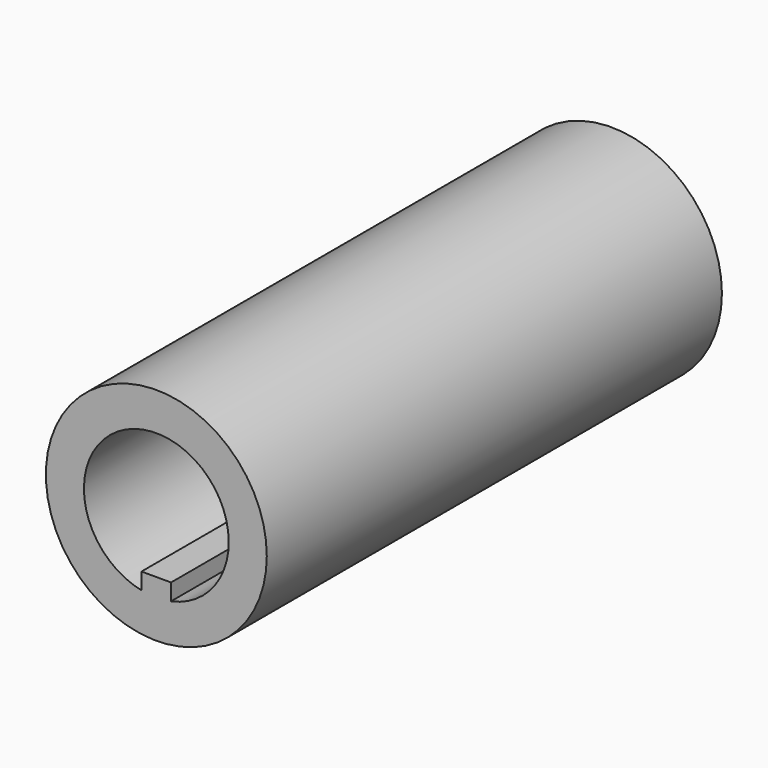
from build123d import *

# Parameters (mm, degrees)
F0_R     = 14.95
F1_DEPTH = 77


# Not quite as in the source:
# - a feature names something its author has since deleted; it is built from what else it names


with BuildPart() as f1:
    # F0 (on Front) → F1 (new body)
    with BuildSketch(Plane.XZ):
        Circle(F0_R)
        with BuildLine():
            ThreePointArc((-1.9898477157, -9.5958587978), (0, 9.8), (1.9898477157, -9.5958587978))
            Line((1.9898477157, -9.5958587978), (1.9898477157, -7.35))
            Line((1.9898477157, -7.35), (-2.0101522843, -7.35))
            Line((-2.0101522843, -7.35), (-1.9898477157, -9.5958587978))
        make_face(mode=Mode.SUBTRACT)
    extrude(amount=F1_DEPTH)


solid = f1.part
